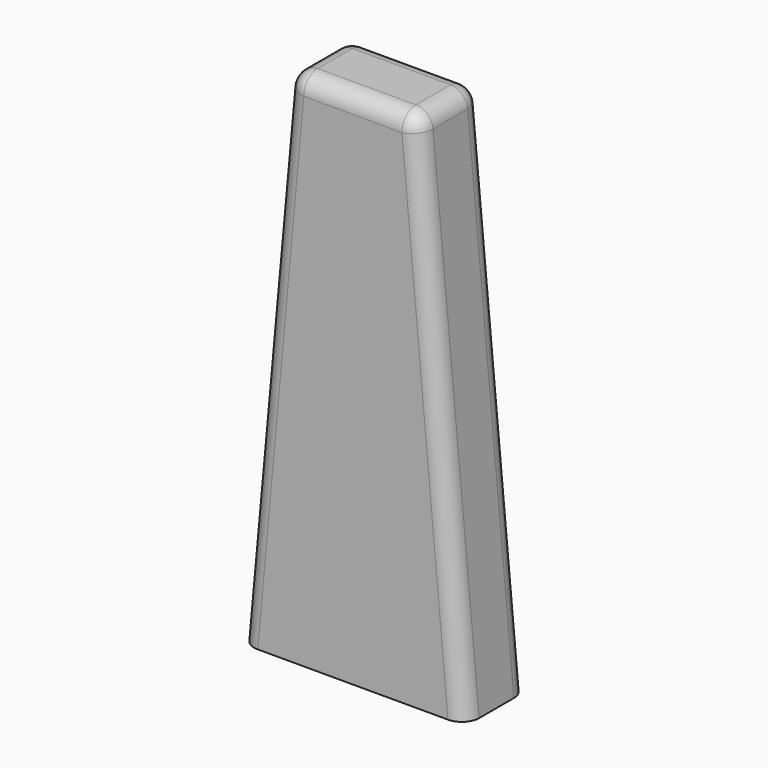
from build123d import *

# Parameters (mm, degrees)
F1_DEPTH = 2.25
F2_R     = 1
F3_T     = 1


# Not quite as in the source:
# - a shell that OpenCascade refuses in one call is made with other operations: the cavity is built on its own and cut out


with BuildPart() as f1:
    # F0 (on Front) → F1 (new body, symmetric)
    with BuildSketch(Plane.XZ):
        Polygon((-3.75, 30), (-6.5, 0), (6.5, 0), (3.75, 30), align=None)
    extrude(amount=F1_DEPTH, both=True)

    # F2
    f2_edges = [f1.edges().sort_by_distance(p)[0] for p in [
        (-3.75, 0, 30),
        (3.75, 0, 30),
        (5.125, -2.25, 15),
        (0, -2.25, 30),
        (-5.125, -2.25, 15),
        (-5.125, 2.25, 15),
        (5.125, 2.25, 15),
        (0, 2.25, 30),
    ]]
    fillet(f2_edges, radius=F2_R)

    # F3: shell of thickness 1, made by hand


with BuildPart() as f3_core1:
    # F3_t2: copy of F1
    add(f1.part)

    # the walls: a layer under each face that stays
    f3_faces = [f3_core1.faces().sort_by_distance(p)[0] for p in [
        (-5.1666494856, 0, 14.5456419748),
        (0, 2.25, 14.5),
        (0, -2.25, 14.5),
        (5.1666494856, 0, 14.5456419748),
        (0, 0, 30),
    ]]
    thicken(f3_faces, amount=-F3_T, mode=Mode.SUBTRACT)


with BuildPart() as f1_1:
    add(f1.part)

    # what is left inside the walls is the cavity
    f3_cavity = [f3_core1.part.solids().sort_by_distance(p)[0] for p in [
        (0, -1.24, 9.666667),
    ]]
    add(f3_cavity, mode=Mode.SUBTRACT)


solid = f1_1.part
